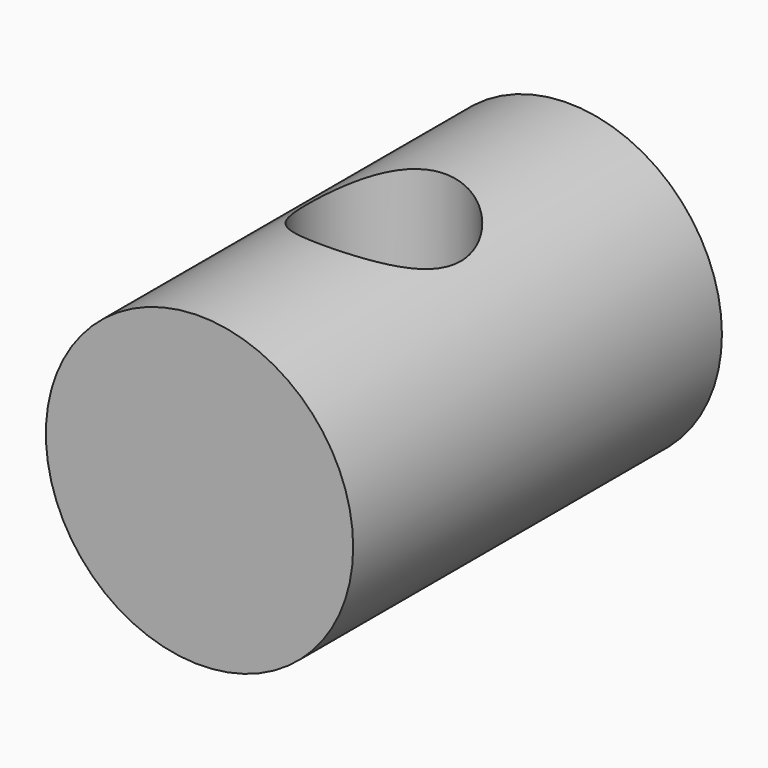
from build123d import *

# Parameters (mm, degrees)
F0_R     = 12.7
F1_DEPTH = 38.1
F2_R     = 6.35
F3_DEPTH = 12.7


# Not quite as in the source:
# - a feature names something its author has since deleted; it is built from what else it names


with BuildPart() as f1:
    # F0 (on Front) → F1 (new body)
    with BuildSketch(Plane.XZ):
        Circle(F0_R)
    extrude(amount=F1_DEPTH)

    # F2 (on Top) → F3 (cut)
    with BuildSketch(Plane.XY):
        with Locations((0, -19.05)):
            Circle(F2_R)
    extrude(amount=F3_DEPTH, mode=Mode.SUBTRACT)


solid = f1.part
